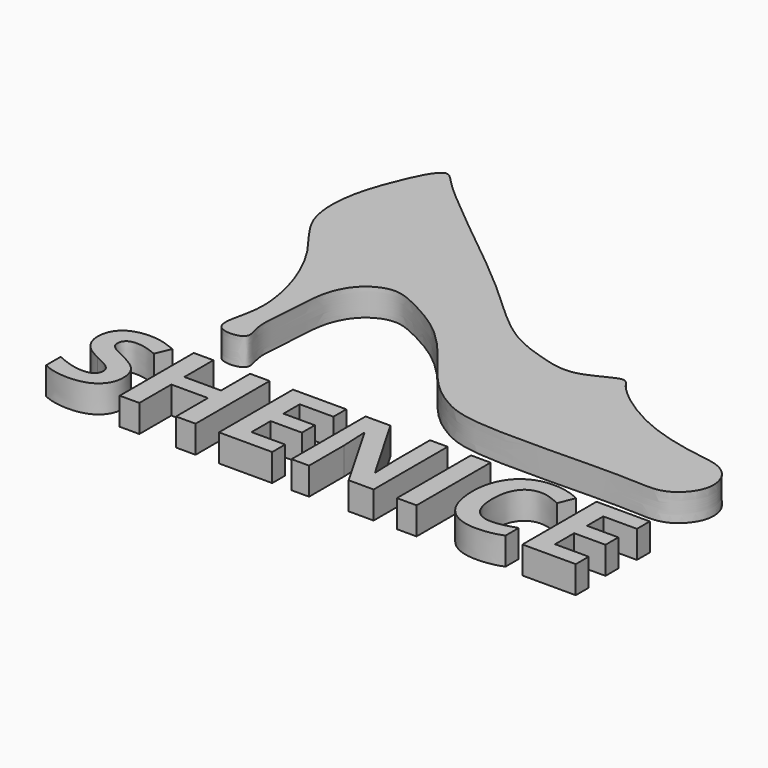
from build123d import *

# Parameters (mm, degrees)
F1_DEPTH     = 2
F2_TEXT_SIZE = 9.472009472
F3_DEPTH     = 2


# Not quite as in the source:
# - Text() gives the source's letters only with a copy of the font that has no kerning and outlines rounded to 1/6400 em; it was checked with that copy


with BuildPart() as f1:
    # F0 (on Top) → F1 (new body)
    with BuildSketch(Plane.XY):
        with BuildLine():
            add(Edge.make_bspline(
                [(7.0431544445, 1.4348232653), (6.7323777753, 1.1198072105), (4.5357758795, 0.9895015657), (5.635497105, 4.0528671391), (5.4553751482, 6.4633008626), (4.8105388603, 8.9923661179), (3.3061654569, 12.127347954), (0.7470681242, 14.8914943733), (0.7064415453, 18.3959851994), (1.5208275824, 21.183775992), (3.2168137409, 24.9590543224), (4.4710712808, 23.3631049782), (8.4554382553, 20.0434975116), (14.6980610817, 15.1183869871), (18.6745252188, 11.0519435636), (21.9691272976, 9.9275960848), (24.6595142466, 9.2062030096), (27.3779085514, 11.1582505065), (27.8628735111, 9.8650956363), (31.6742159638, 7.030678151), (36.2405003991, 6.1166593394), (38.1625742583, 5.9072985308), (39.3131398491, 4.8859533072), (39.5576458137, 3.2378341112), (38.6113687264, 1.8739188622), (37.2362492335, 1.1239792509), (34.3523779336, 1.5431059513), (23.78448994, 0.9648059558), (21.2062037056, 2.2198753354), (19.2883147645, 3.557775883), (17.0516060195, 6.6562200656), (14.7838604463, 9.0999164654), (11.9607956901, 10.6731237757), (10.1079585494, 11.4008888115), (8.1578517448, 10.4357314058), (7.0869951265, 8.2955692024), (7.140159771, 5.4677150171), (6.7012529967, 2.8532219941), (7.3131911476, 1.7085436094), (7.0431544445, 1.4348232653)],
                knots=[0, 0, 0, 0, 0.0207821507, 0.0456968308, 0.0712099009, 0.0965445225, 0.1261853933, 0.1567030208, 0.1850980239, 0.2139474867, 0.2427304626, 0.2597659419, 0.2960925061, 0.3421027541, 0.3798367406, 0.408713914, 0.4350982386, 0.4612187355, 0.4760918054, 0.5104129845, 0.5453784261, 0.566863757, 0.5854052683, 0.6050415905, 0.6248896635, 0.6432421094, 0.6705402073, 0.7222573093, 0.7490159112, 0.7723518483, 0.8032691191, 0.832844771, 0.8611545599, 0.8828811462, 0.9048375042, 0.9287700916, 0.9557205423, 0.9819421983, 1, 1, 1, 1], degree=3))
        make_face()
    extrude(amount=F1_DEPTH)


with BuildPart() as f3:
    # F2 (on Top) → F3 (new body)
    with BuildSketch(Plane.XY):
        with Locations((0, -8.7774778625)):
            Text('SHENICE', F2_TEXT_SIZE, font='Open Sans', font_style=FontStyle.BOLD, text_align=(TextAlign.LEFT, TextAlign.BOTTOM))
    extrude(amount=F3_DEPTH)


solid = Compound([f1.part, f3.part])
